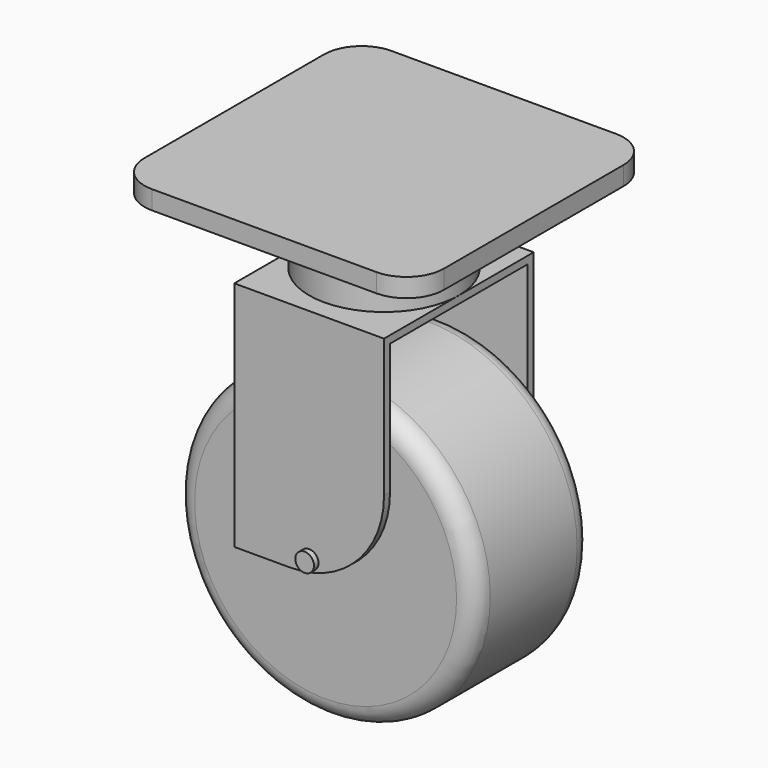
from build123d import *
from build123d import SkipClean  # not in build123d's __all__

# Parameters (mm, degrees)
F0_W      = 80
F0_H      = 5
F1_DEPTH  = 40
F3_DEPTH  = 20
F5_DEPTH  = 2
F6_W      = 40
F6_H      = 2
F7_DEPTH  = 60
F8_R      = 2.5
F9_DEPTH  = 3.5
F10_R     = 40
F10_R_2   = 2.5
F11_DEPTH = 19.5
F13_R     = 5
F14_R     = 10
F15_R     = 25
F16_R     = 25


with BuildPart() as f1:
    # F0 (on Front) → F1 (new body)
    with BuildSketch(Plane.XZ):
        with Locations((0, 40.0008145292)):
            Rectangle(F0_W, F0_H)
    extrude(amount=-F1_DEPTH)

    # F2 (on face) → F3 (join)
    with BuildSketch(Plane(origin=(0, 0, 37.5008145292), x_dir=(1, 0, 0), z_dir=(0, 0, -1))):
        with BuildLine():
            Line((20, 0), (-20, 0))
            ThreePointArc((-20, 0), (0, -20), (20, 0))
        make_face()
    extrude(amount=F3_DEPTH)

    # F4 (on face) → F5 (join)
    with BuildSketch(Plane(origin=(0, 0, 17.5008145292), x_dir=(1, 0, 0), z_dir=(0, 0, -1))):
        with BuildLine():
            ThreePointArc((20, 0), (0, -20), (-20, 0))
            Line((-20, 0), (-20, -25))
            Line((-20, -25), (20, -25))
            Line((20, -25), (20, 0))
        make_face()
        with BuildLine():
            Line((20, 0), (-20, 0))
            ThreePointArc((-20, 0), (0, -20), (20, 0))
        make_face()
    extrude(amount=F5_DEPTH)

    # F6 (on face) → F7 (join)
    with BuildSketch(Plane(origin=(0, 0, 15.5008145292), x_dir=(1, 0, 0), z_dir=(0, 0, -1))):
        with Locations((0, -24)):
            Rectangle(F6_W, F6_H)
    extrude(amount=F7_DEPTH)

    # F8 (on face) → F9 (join, symmetric)
    with BuildSketch(Plane.XZ.offset(-23)):
        with Locations((0, -40.9991854708)):
            Circle(F8_R)
    extrude(amount=F9_DEPTH, both=True)

    # F10 (on face) → F11 (join, through all)
    with BuildSketch(Plane.XZ.offset(-19.5)):
        with Locations((0, -40.9991854708)):
            Circle(F10_R)
        with Locations((0, -40.9991854708)):
            Circle(F10_R_2, mode=Mode.SUBTRACT)
        with Locations((0, -40.9991854708)):
            Circle(F10_R_2)
    extrude(amount=F11_DEPTH)

    # F12: F1 across face


with BuildPart() as f1_1:
    add(f1.part, clean=False)
    with SkipClean():  # cleaning this boolean's faces spoils the solid; the shape is the same uncleaned
        add(f1.part.mirror(Plane(origin=(0, 0, 30.7195645292), x_dir=(1, 0, 0), z_dir=(0, -1, 0))), clean=False)

    # F13
    f13_edges = [f1_1.edges().sort_by_distance(p)[0] for p in [
        (-40, 19.5, -40.999185),
        (-40, -19.5, -40.999185),
    ]]
    fillet(f13_edges, radius=F13_R)

    # F14
    f14_edges = [f1_1.edges().sort_by_distance(p)[0] for p in [
        (40, -40, 40.000815),
        (-40, -40, 40.000815),
        (-40, 40, 40.000815),
        (40, 40, 40.000815),
    ]]
    fillet(f14_edges, radius=F14_R)

    # F15
    f15_edges = [f1_1.edges().sort_by_distance(p)[0] for p in [
        (20, 24, -44.499185),
    ]]
    fillet(f15_edges, radius=F15_R)

    # F16
    f16_edges = [f1_1.edges().sort_by_distance(p)[0] for p in [
        (20, -24, -44.499185),
    ]]
    fillet(f16_edges, radius=F16_R)


solid = f1_1.part
